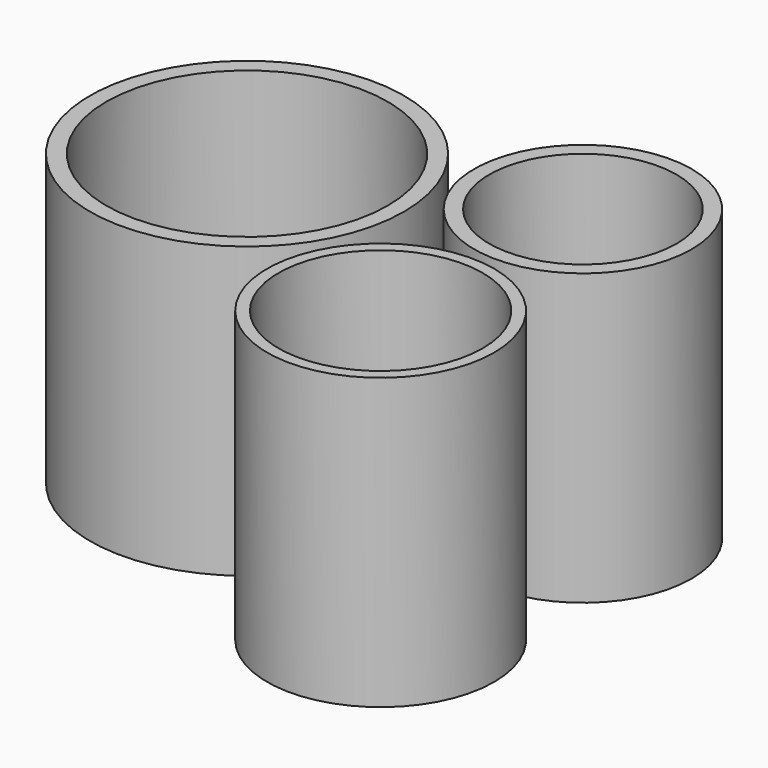
from build123d import *

# Parameters (mm, degrees)
F0_R        = 32.5
F1_DEPTH    = 60
F0_R_2      = 22.5
F0_R_3      = 23.5
F2_R        = 19
F3_DEPTH    = 60
F5_R        = 29.125
F5_R_2      = 19.375
F5_R_3      = 21.125
F6_DEPTH    = 30
F7_S5_R     = 29.125
F7_T6_DEPTH = 50


# Not quite as in the source:
# - a fillet or chamfer that OpenCascade refuses, or shapes differently, is made with other operations: its cross-section is extruded or revolved along the edge and cut away or added


with BuildPart() as f1:
    # F0 (on Top) → F1 (new body)
    with BuildSketch(Plane.XY):
        with Locations((-29.2519945651, 19.268617034)):
            Circle(F0_R)
    extrude(amount=F1_DEPTH)


with BuildPart() as f1b:
    # F0 (on Top) → F1, piece 2 (new body)
    with BuildSketch(Plane.XY):
        with Locations((25.2509750426, 38.0198201165)):
            Circle(F0_R_2)
    extrude(amount=F1_DEPTH)


with BuildPart() as f1c:
    # F0 (on Top) → F1, piece 3 (new body)
    with BuildSketch(Plane.XY):
        with Locations((21.9174157828, -10.1318648085)):
            Circle(F0_R_3)
    extrude(amount=F1_DEPTH)


with BuildPart() as f3_tool:
    # F2 (on Top) → F3 (new body, through all)
    with BuildSketch(Plane.XY):
        with Locations((-29.2519945651, 19.268617034)):
            Circle(F2_R)
        with Locations((25.2509750426, 38.0198201165)):
            Circle(F2_R)
        with Locations((21.9174157828, -10.1318648085)):
            Circle(F2_R)
    extrude(amount=F3_DEPTH)


with BuildPart() as f1_1:
    add(f1.part)

    # F3: cut by f3_tool
    add(f3_tool.part, mode=Mode.SUBTRACT)


with BuildPart() as f1b_1:
    add(f1b.part)

    # F3: cut by f3_tool
    add(f3_tool.part, mode=Mode.SUBTRACT)


with BuildPart() as f1c_1:
    add(f1c.part)

    # F3: cut by f3_tool
    add(f3_tool.part, mode=Mode.SUBTRACT)


with BuildPart() as f6_tool:
    # F5 (on offset) → F6 (new body)
    with BuildSketch(Plane.XY.offset(60)):
        with Locations((-29.2519945651, 19.268617034)):
            Circle(F5_R)
        with Locations((25.2509750426, 38.0198201165)):
            Circle(F5_R_2)
        with Locations((21.9174157828, -10.1318648085)):
            Circle(F5_R_3)
    extrude(amount=-F6_DEPTH)


with BuildPart() as f1_2:
    add(f1_1.part)

    # F6: cut by f6_tool
    add(f6_tool.part, mode=Mode.SUBTRACT)

    # F7: chamfer of 15 on 1 edges, made by hand


with BuildPart() as f1b_2:
    add(f1b_1.part)

    # F6: cut by f6_tool
    add(f6_tool.part, mode=Mode.SUBTRACT)


with BuildPart() as f1c_2:
    add(f1c_1.part)

    # F6: cut by f6_tool
    add(f6_tool.part, mode=Mode.SUBTRACT)


with BuildPart() as f7_tool2:
    # F7_s3 → F7_t4 (revolve)
    with BuildSketch(Plane.XZ.offset(-19.268617034)):
        Polygon((-10.2519945651, 15), (4.7480054349, 30), (-10.2519945651, 30), align=None)
    revolve(axis=Axis((-29.2519945651, 19.268617034, 30), (0, 0, -1)))

    # F7_s5 → F7_t6 (intersect, symmetric)
    with BuildSketch(Plane.XY.offset(22.5)):
        with Locations((-29.2519945651, 19.268617034)):
            Circle(F7_S5_R)
    extrude(amount=F7_T6_DEPTH, both=True, mode=Mode.INTERSECT)


with BuildPart() as f1_3:
    add(f1_2.part)

    # F7_t1: cut F7_tool2
    add(f7_tool2.part, mode=Mode.SUBTRACT)


solid = Compound([f1b_2.part, f1c_2.part, f1_3.part])
